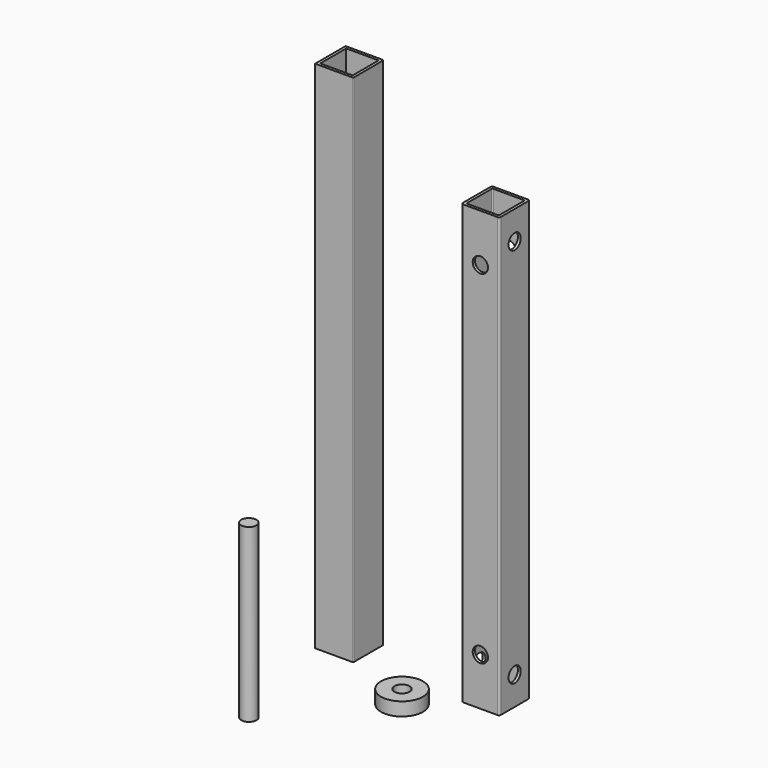
from build123d import *

# Parameters (mm, degrees)
F1_R      = 11
F1_R_2    = 4
F2_DEPTH  = 7
F3_W      = 20
F3_H      = 20
F4_DEPTH  = 270
F5_R      = 0.5
F6_T      = -1.5
F7_W      = 20
F7_H      = 20
F8_DEPTH  = 230
F9_R      = 1
F10_T     = -1.5
F12_D     = 8
F14_D     = 8
F15_R     = 4
F16_DEPTH = 90
F17_R     = 0.5


with BuildPart() as f2:
    # F1 (on Top) → F2 (new body)
    with BuildSketch(Plane.XY):
        Circle(F1_R)
        Circle(F1_R_2, mode=Mode.SUBTRACT)
    extrude(amount=F2_DEPTH)


with BuildPart() as f4:
    # F3 (on Top) → F4 (new body)
    with BuildSketch(Plane.XY):
        with Locations((-48.7633477896, 26.4656734091)):
            Rectangle(F3_W, F3_H)
    extrude(amount=F4_DEPTH)

    # F5
    f5_edges = [f4.edges().sort_by_distance(p)[0] for p in [
        (-38.763348, 36.465673, 135),
        (-38.763348, 16.465673, 135),
    ]]
    fillet(f5_edges, radius=F5_R)

    # F6
    f6_openings = [f4.faces().sort_by_distance(p)[0] for p in [
        (-48.766001, 26.465673, 270),
        (-48.766001, 26.465673, 0),
    ]]
    offset(amount=F6_T, openings=f6_openings)


with BuildPart() as f8:
    # F7 (on Top) → F8 (new body)
    with BuildSketch(Plane.XY):
        with Locations((27.6069855317, 26.8707028835)):
            Rectangle(F7_W, F7_H)
    extrude(amount=F8_DEPTH)

    # F9
    f9_edges = [f8.edges().sort_by_distance(p)[0] for p in [
        (37.606986, 36.870703, 115),
        (17.606986, 36.870703, 115),
        (37.606986, 16.870703, 115),
        (17.606986, 16.870703, 115),
    ]]
    fillet(f9_edges, radius=F9_R)

    # F10
    f10_openings = [f8.faces().sort_by_distance(p)[0] for p in [
        (27.606986, 26.870703, 230),
        (27.606986, 26.870703, 0),
    ]]
    offset(amount=F10_T, openings=f10_openings)

    # F12 (through all)
    with Locations(Plane.YZ.offset(37.6069855317)):
        with Locations((26.8707028835, 15), (26.8707028835, 215)):
            Hole(F12_D / 2)

    # F14 (through all)
    with Locations(Plane(origin=(0, 36.8707028835, 0), x_dir=(-1, 0, 0), z_dir=(0, 1, 0))):
        with Locations((-27.6069855317, 205), (-27.6069855317, 25)):
            Hole(F14_D / 2)

    # F17
    f17_edges = [f8.edges().sort_by_distance(p)[0] for p in [
        (36.106986, 35.370703, 115),
        (19.106986, 35.370703, 115),
        (36.106986, 18.370703, 115),
        (19.106986, 18.370703, 115),
    ]]
    fillet(f17_edges, radius=F17_R)


with BuildPart() as f16:
    # F15 (on Top) → F16 (new body)
    with BuildSketch(Plane.XY):
        with Locations((-41.6371822357, -48.3863502741)):
            Circle(F15_R)
    extrude(amount=F16_DEPTH)


solid = Compound([f2.part, f4.part, f8.part, f16.part])
